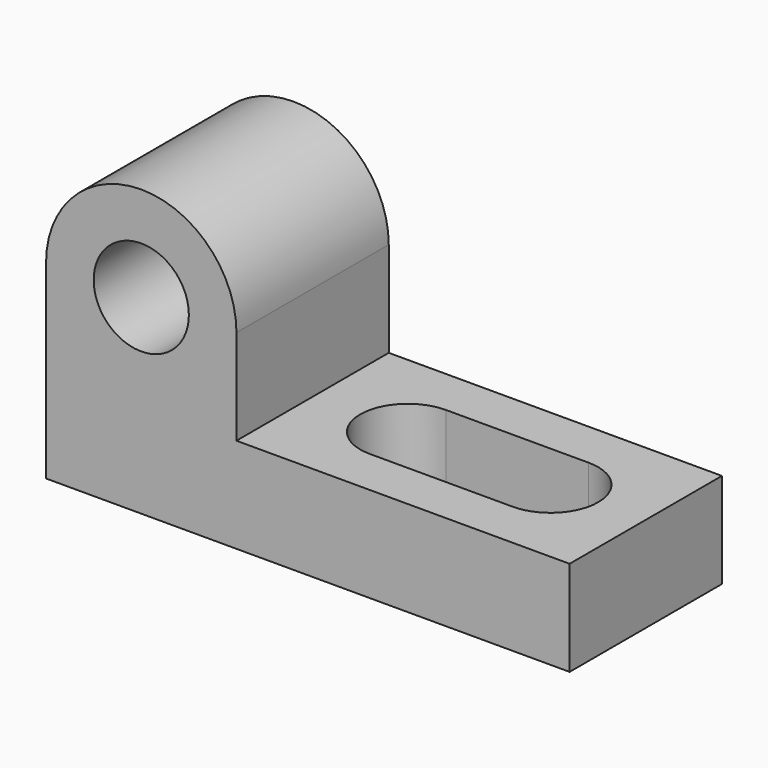
from build123d import *

# Parameters (mm, degrees)
F1_DEPTH = 25.4
F4_DEPTH = 12.7
F2_R     = 6.35
F5_DEPTH = 25.4


# Not quite as in the source:
# - ends of sketch curves that miss each other by under 0.0002 mm in the source are joined


with BuildPart() as f1:
    # F0 (on Front) → F1 (new body)
    with BuildSketch(Plane.XZ):
        Polygon((-46.4223937518, 20.1214007731), (-71.8223937518, 20.1214007731), (-71.8223937518, -17.9785992269), (-1.9723937518, -17.9785992269), (-1.9723937518, -5.2785992269), (-46.4223937518, -5.2785992269), align=None)
    extrude(amount=F1_DEPTH)

    # F3 (on face) → F4 (cut)
    with BuildSketch(Plane.XY.offset(-5.2785992269)):
        with BuildLine():
            ThreePointArc((-8.3223937518, -12.6999999235), (-10.1822656913, -8.2098718629), (-14.6723937518, -6.3499999235))
            ThreePointArc((-14.6723937518, -6.3499999235), (-21.0223937518, -12.6999999235), (-14.6723937518, -19.0499999235))
            ThreePointArc((-14.6723937518, -19.0499999235), (-10.1822656913, -17.190127984), (-8.3223937518, -12.6999999235))
        make_face()
        with BuildLine():
            ThreePointArc((-33.7223937518, -6.3499998086), (-29.2322656913, -8.2098717481), (-27.3723937518, -12.6999998086))
            ThreePointArc((-27.3723937518, -12.6999998086), (-29.2322656913, -17.1901278692), (-33.7223937518, -19.0499998086))
            Line((-33.7223937518, -19.0499998086), (-14.6723937518, -19.0499998086))
            ThreePointArc((-14.6723937518, -19.0499998086), (-21.0223937518, -12.6999999235), (-14.6723937518, -6.3499999235))
            Line((-14.6723937518, -6.3499999235), (-33.7223937518, -6.3499998086))
        make_face()
        with BuildLine():
            ThreePointArc((-33.7223937518, -19.0499998086), (-29.2322656913, -17.1901278692), (-27.3723937518, -12.6999998086))
            ThreePointArc((-27.3723937518, -12.6999998086), (-29.2322656913, -8.2098717481), (-33.7223937518, -6.3499998086))
            ThreePointArc((-33.7223937518, -6.3499998086), (-40.0723937518, -12.6999998086), (-33.7223937518, -19.0499998086))
        make_face()
    extrude(amount=-F4_DEPTH, mode=Mode.SUBTRACT)

    # F2 (on face) → F5 (cut)
    with BuildSketch(Plane.XZ.offset(25.4)):
        with Locations((-59.1223937518, 7.4214007731)):
            Circle(F2_R)
        with BuildLine():
            ThreePointArc((-71.8223937518, 7.4214007731), (-59.1223937518, 20.1043120223), (-46.4223937518, 7.4214007731))
            Line((-46.4223937518, 7.4214007731), (-46.4223937518, 20.1214007731))
            Line((-46.4223937518, 20.1214007731), (-71.8223937518, 20.1214007731))
            Line((-71.8223937518, 20.1214007731), (-71.8223937518, 7.4214007731))
        make_face()
    extrude(amount=-F5_DEPTH, mode=Mode.SUBTRACT)


solid = f1.part
